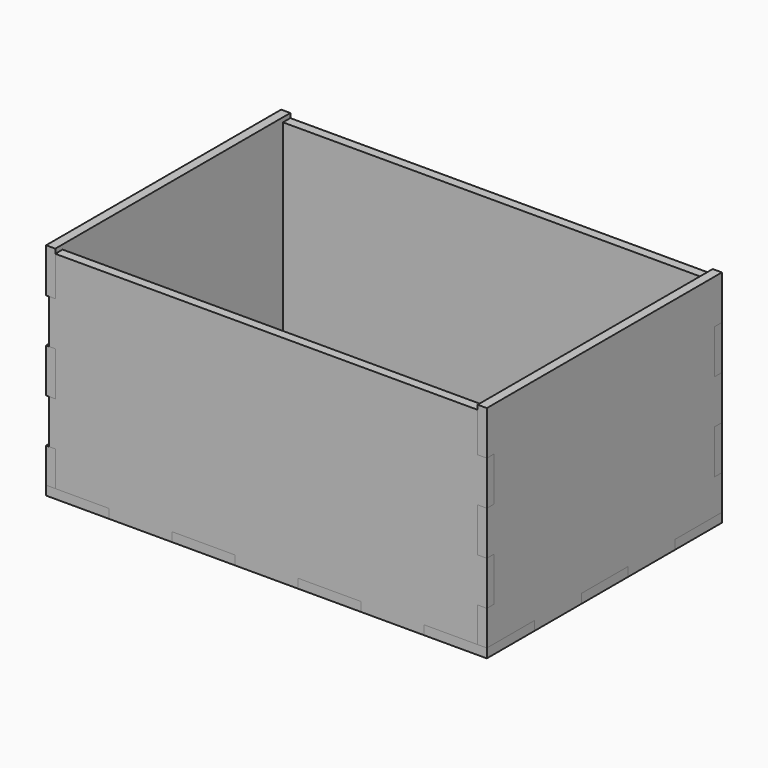
from build123d import *

# Parameters (mm, degrees)
F0_W     = 3.175
F0_H     = 17.074
F0_W_2   = 18.5964285714
F0_H_2   = 3.175
F0_W_3   = 21.7714285714
F0_H_3   = 20.249
F0_H_4   = 17.429
F0_H_5   = 2.82
F1_DEPTH = 3.175
F2_W     = 3.175
F2_H     = 15.24
F2_H_2   = 12.065
F3_DEPTH = 3.175
F7_DEPTH = 3.175


with BuildPart() as f1:
    # F0 (on Top) → F1 (new body)
    with BuildSketch(Plane.XY):
        with Locations((-74.6125, 39.088)):
            Rectangle(F0_W, F0_H)
        with Locations((-63.7267857143, 49.2125)):
            Rectangle(F0_W_2, F0_H_2)
        with Locations((-74.6125, 49.2125)):
            Rectangle(F0_W, F0_H_2)
        with Locations((-21.7714285714, 49.2125)):
            Rectangle(F0_W_3, F0_H_2)
        Polygon((73.025, 30.551), (73.025, 47.625), (54.4285714286, 47.625), (32.6571428571, 47.625), (10.8857142857, 47.625), (-10.8857142857, 47.625), (-32.6571428571, 47.625), (-54.4285714286, 47.625), (-73.025, 47.625), (-73.025, 30.551), (-73.025, 10.302), (-73.025, -9.947), (-73.025, -30.196), (-73.025, -47.625), (-54.4285714286, -47.625), (-32.6571428571, -47.625), (-10.8857142857, -47.625), (10.8857142857, -47.625), (32.6571428571, -47.625), (54.4285714286, -47.625), (73.025, -47.625), (73.025, -30.196), (73.025, -9.947), (73.025, 10.302), align=None)
        with Locations((21.7714285714, 49.2125)):
            Rectangle(F0_W_3, F0_H_2)
        with Locations((63.7267857143, 49.2125)):
            Rectangle(F0_W_2, F0_H_2)
        with Locations((74.6125, 49.2125)):
            Rectangle(F0_W, F0_H_2)
        with Locations((74.6125, 39.088)):
            Rectangle(F0_W, F0_H)
        with Locations((74.6125, 0.1775)):
            Rectangle(F0_W, F0_H_3)
        with Locations((74.6125, -38.9105)):
            Rectangle(F0_W, F0_H_4)
        with Locations((74.6125, -49.035)):
            Rectangle(F0_W, F0_H_5)
        Polygon((73.025, -50.445), (73.025, -47.625), (54.4285714286, -47.625), (54.4285714286, -50.8), (73.025, -50.8), (76.2, -50.8), (76.2, -50.445), align=None)
        with Locations((21.7714285714, -49.2125)):
            Rectangle(F0_W_3, F0_H_2)
        with Locations((-21.7714285714, -49.2125)):
            Rectangle(F0_W_3, F0_H_2)
        Polygon((-54.4285714286, -50.8), (-54.4285714286, -47.625), (-73.025, -47.625), (-73.025, -50.445), (-76.2, -50.445), (-76.2, -50.8), (-73.025, -50.8), align=None)
        with Locations((-74.6125, -49.035)):
            Rectangle(F0_W, F0_H_5)
        with Locations((-74.6125, -38.9105)):
            Rectangle(F0_W, F0_H_4)
        with Locations((-74.6125, 0.1775)):
            Rectangle(F0_W, F0_H_3)
    extrude(amount=F1_DEPTH)


with BuildPart() as f3:
    # F2 (on face) → F3 (new body)
    with BuildSketch(Plane.YZ.offset(76.2)):
        Polygon((-30.196, 3.175), (-30.196, 0), (47.625, 0), (47.625, 15.24), (47.625, 30.48), (47.625, 45.72), (47.625, 60.96), (47.625, 76.2), (-47.625, 76.2), (-47.625, 60.96), (-47.625, 45.72), (-47.625, 30.48), (-47.625, 15.24), (-47.625, 3.175), align=None)
        with Locations((-49.2125, 68.58)):
            Rectangle(F2_W, F2_H)
        with Locations((-49.2125, 38.1)):
            Rectangle(F2_W, F2_H)
        with Locations((-49.2125, 9.2075)):
            Rectangle(F2_W, F2_H_2)
        with Locations((49.2125, 68.58)):
            Rectangle(F2_W, F2_H)
        with Locations((49.2125, 38.1)):
            Rectangle(F2_W, F2_H)
        with Locations((49.2125, 7.62)):
            Rectangle(F2_W, F2_H)
    extrude(amount=-F3_DEPTH)


with BuildPart() as f4_1:
    # F4: instance of F3
    add(f3.part.mirror(Plane.YZ))

    # F5: cut F1
    add(f1.part, mode=Mode.SUBTRACT)


with BuildPart() as f3_1:
    add(f3.part)

    # F5: cut F1
    add(f1.part, mode=Mode.SUBTRACT)


with BuildPart() as f7:
    # F6 (on face) → F7 (new body)
    with BuildSketch(Plane(origin=(0, 50.8, 0), x_dir=(-1, 0, 0), z_dir=(0, 1, 0))):
        Polygon((75.1678422093, 74.6399760246), (-76.2, 74.6399760246), (-76.2, 3.175), (-54.4285714286, 3.175), (-54.4285714286, 0), (75.1678422093, 0), align=None)
    extrude(amount=-F7_DEPTH)


with BuildPart() as f8_1:
    # F8: instance of F7
    add(f7.part.mirror(Plane.XZ))

    # F9: cut F3, F1, F4_1
    add(f3_1.part, mode=Mode.SUBTRACT)
    add(f1.part, mode=Mode.SUBTRACT)
    add(f4_1.part, mode=Mode.SUBTRACT)


with BuildPart() as f7_1:
    add(f7.part)

    # F9: cut F3, F1, F4_1
    add(f3_1.part, mode=Mode.SUBTRACT)
    add(f1.part, mode=Mode.SUBTRACT)
    add(f4_1.part, mode=Mode.SUBTRACT)


solid = Compound([f1.part, f4_1.part, f3_1.part, f8_1.part, f7_1.part])
